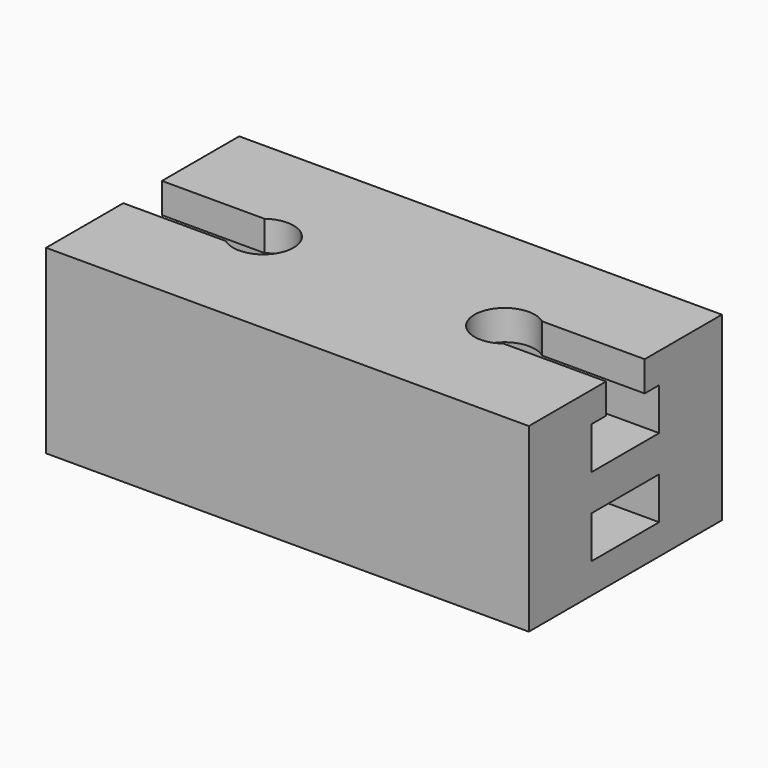
from build123d import *

# Parameters (mm, degrees)
F0_W            = 40
F0_H            = 20
F1_DEPTH        = 15
F2_R            = 2.5
F3_DEPTH        = 15.001
F4_W            = 7
F4_H            = 3.5
F5_DEPTH        = 14.5
F6_W            = 4
F6_H            = 2.5
F7_DEPTH        = 12.5
F7_COPIES_COUNT = 2
F7_COPIES_PITCH = 31.5
F8_T1_DEPTH     = 2.5
F9_T4_DEPTH     = 2.5
F9_S5_R         = 2.5
F9_T6_DEPTH     = 4


# Not quite as in the source:
# - a fillet or chamfer that OpenCascade refuses, or shapes differently, is made with other operations: its cross-section is extruded or revolved along the edge and cut away or added
# - a pattern or mirror of a feature is missing from the dataset's text; its kind, count and spacing are read off the source's solid


with BuildPart() as f1:
    # F0 (on Top) → F1 (new body)
    with BuildSketch(Plane.XY):
        Rectangle(F0_W, F0_H)
    extrude(amount=F1_DEPTH)

    # F2 (on face) → F3 (cut, through all)
    with BuildSketch(Plane.XY.offset(15)):
        with Locations((-10, 0)):
            Circle(F2_R)
        with Locations((10, 0)):
            Circle(F2_R)
    extrude(amount=-F3_DEPTH, mode=Mode.SUBTRACT)

    # F4 (on face) → F5 (cut)
    with BuildSketch(Plane(origin=(-20, 0, 0), x_dir=(0, -1, 0), z_dir=(-1, 0, 0))):
        with Locations((0, 4.25)):
            Rectangle(F4_W, F4_H)
        with Locations((0, 10.75)):
            Rectangle(F4_W, F4_H)
    f5 = extrude(amount=-F5_DEPTH, mode=Mode.SUBTRACT)

    # F5_copies: F5 across plane
    add(f5.mirror(Plane(origin=(0, 0, 0), x_dir=(0, 0, 1), z_dir=(1, 0, 0))), mode=Mode.SUBTRACT)

    # F6 (on face) → F7 (cut)
    with BuildSketch(Plane(origin=(-20, 0, 0), x_dir=(0, -1, 0), z_dir=(-1, 0, 0))):
        with Locations((0, 13.75)):
            Rectangle(F6_W, F6_H)
    f7 = extrude(amount=-F7_DEPTH, mode=Mode.SUBTRACT)

    # F7_copies: F7 ×2
    with Locations(*[(i * F7_COPIES_PITCH, 0, 0) for i in range(1, F7_COPIES_COUNT)]):
        add(f7, mode=Mode.SUBTRACT)

    # F8: fillet of radius 2.5 on 1 edges, made by hand

    # F8_s2 → F8_t1 (join)
    with BuildSketch(Plane.XY.offset(12.5)):
        with BuildLine():
            ThreePointArc((-8.5, -2), (-7.7639320225, -1.1180339887), (-7.5, 0))
            Line((-7.5, 0), (-7.5, -2))
            Line((-7.5, -2), (-8.5, -2))
        make_face()
    extrude(amount=F8_T1_DEPTH)

    # F9: fillet of radius 2.5 on 1 edges, made by hand


with BuildPart() as f9_tool2:
    # F9_s3 → F9_t4 (new body)
    with BuildSketch(Plane.XY.offset(15)):
        with BuildLine():
            ThreePointArc((-7.5, -0.5), (-8.232233047, 1.267766953), (-10, 2))
            Line((-10, 2), (-7.5, 2))
            Line((-7.5, 2), (-7.5, -0.5))
        make_face()
    extrude(amount=-F9_T4_DEPTH)

    # F9_s5 → F9_t6 (cut, symmetric)
    with BuildSketch(Plane.XY.offset(13.8)):
        with Locations((-10, 0)):
            Circle(F9_S5_R)
    extrude(amount=F9_T6_DEPTH, both=True, mode=Mode.SUBTRACT)


with BuildPart() as f1_1:
    add(f1.part)

    # F9_t1: union F9_tool2
    add(f9_tool2.part)


solid = f1_1.part
